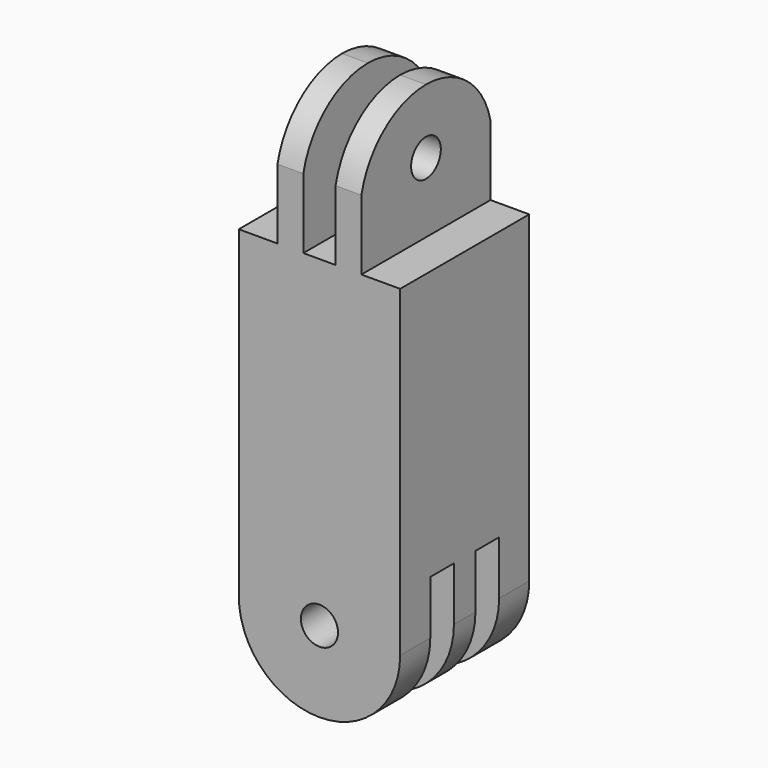
from build123d import *

# Parameters (mm, degrees)
F0_W      = 30
F0_H      = 75
F1_DEPTH  = 30
F4_DEPTH  = 30.001
F2_W      = 30
F2_H      = 5.5
F5_DEPTH  = 25
F3_R      = 3.45
F6_DEPTH  = 30.001
F7_W      = 4.8
F7_H      = 30
F8_DEPTH  = 25
F10_DEPTH = 22.801
F9_R      = 3.45
F11_DEPTH = 22.801


with BuildPart() as f1:
    # F0 (on Right) → F1 (new body)
    with BuildSketch(Plane.YZ):
        Rectangle(F0_W, F0_H)
    extrude(amount=F1_DEPTH)

    # F3 (on face) → F4 (cut, through all)
    with BuildSketch(Plane(origin=(0, 15, 0), x_dir=(-1, 0, 0), z_dir=(0, 1, 0))):
        with BuildLine():
            ThreePointArc((-15, -37.5), (-25.6066017178, -33.1066017178), (-30, -22.5))
            Line((-30, -22.5), (-30, -37.5))
            Line((-30, -37.5), (-15, -37.5))
        make_face()
        with BuildLine():
            ThreePointArc((0, -22.5), (-4.3933982822, -33.1066017178), (-15, -37.5))
            Line((-15, -37.5), (0, -37.5))
            Line((0, -37.5), (0, -22.5))
        make_face()
    extrude(amount=-F4_DEPTH, mode=Mode.SUBTRACT)

    # F2 (on face) → F5 (cut)
    with BuildSketch(Plane(origin=(0, 0, -37.5), x_dir=(1, 0, 0), z_dir=(0, 0, -1))):
        with Locations((15, 5.25)):
            Rectangle(F2_W, F2_H)
        with Locations((15, -5.25)):
            Rectangle(F2_W, F2_H)
    extrude(amount=-F5_DEPTH, mode=Mode.SUBTRACT)

    # F3 (on face) → F6 (cut, through all)
    with BuildSketch(Plane(origin=(0, 15, 0), x_dir=(-1, 0, 0), z_dir=(0, 1, 0))):
        with Locations((-15, -22.5)):
            Circle(F3_R)
    extrude(amount=-F6_DEPTH, mode=Mode.SUBTRACT)

    # F7 (on face) → F8 (join)
    with BuildSketch(Plane.XY.offset(37.5)):
        with Locations((9.6, 0)):
            Rectangle(F7_W, F7_H)
        with Locations((20.4, 0)):
            Rectangle(F7_W, F7_H)
    extrude(amount=F8_DEPTH)

    # F9 (on face) → F10 (cut, through all)
    with BuildSketch(Plane(origin=(7.2, 0, 0), x_dir=(0, -1, 0), z_dir=(-1, 0, 0))):
        with BuildLine():
            ThreePointArc((-15, 50.5), (-9.6046863561, 59.1308579452), (0, 62.5))
            Line((0, 62.5), (-15, 62.5))
            Line((-15, 62.5), (-15, 50.5))
        make_face()
        with BuildLine():
            ThreePointArc((0, 62.5), (9.6046863561, 59.1308579452), (15, 50.5))
            Line((15, 50.5), (15, 62.5))
            Line((15, 62.5), (0, 62.5))
        make_face()
    extrude(amount=-F10_DEPTH, mode=Mode.SUBTRACT)

    # F9 (on face) → F11 (cut, through all)
    with BuildSketch(Plane(origin=(7.2, 0, 0), x_dir=(0, -1, 0), z_dir=(-1, 0, 0))):
        with Locations((0, 50.5)):
            Circle(F9_R)
    extrude(amount=-F11_DEPTH, mode=Mode.SUBTRACT)


solid = f1.part
